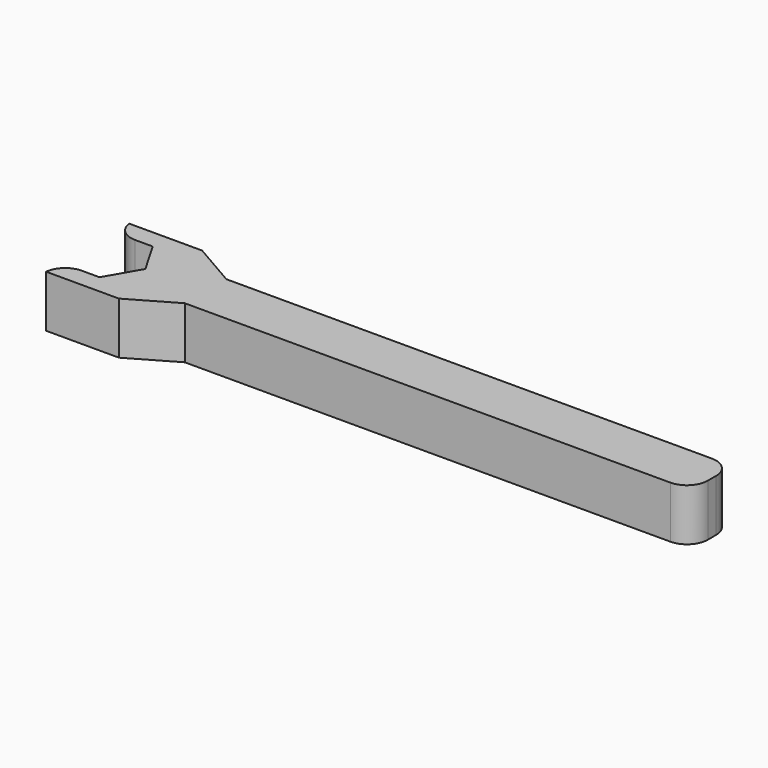
from build123d import *

# Parameters (mm, degrees)
F1_DEPTH    = 2.5
F2_T1_DEPTH = 14.9498743711
F2_T3_DEPTH = 15


# Not quite as in the source:
# - a fillet or chamfer that OpenCascade refuses, or shapes differently, is made with other operations: its cross-section is extruded or revolved along the edge and cut away or added


with BuildPart() as f1:
    # F0 (on Top) → F1 (new body, symmetric)
    with BuildSketch(Plane.XY):
        Polygon((1.8475208614, 3.2), (3.6950417228, 0), (1.8475208614, -3.2), (-1.8475208614, -3.2), (-1.8475208614, -5), (5.1524791386, -5), (9.4826061575, -2.5), (58.1524791386, -2.5), (58.1524791386, 2.5), (9.4826061575, 2.5), (5.1524791386, 5), (-1.8475208614, 5), (-1.8475208614, 3.2), align=None)
    extrude(amount=F1_DEPTH, both=True)

    # F2: fillet of radius 2 on 4 edges, made by hand

    # F2_s2 → F2_t1 (cut)
    with BuildSketch(Plane.XY.offset(-7.4749371855)):
        with BuildLine():
            ThreePointArc((-1.8475208614, 5), (-1.1991867737, 3.7167603026), (0.1424540128, 3.2))
            Line((0.1424540128, 3.2), (-1.8475208614, 3.2))
            Line((-1.8475208614, 3.2), (-1.8475208614, 5))
        make_face()
        with BuildLine():
            ThreePointArc((-1.8475208614, -5), (-1.1991867737, -3.7167603026), (0.1424540128, -3.2))
            Line((0.1424540128, -3.2), (-1.8475208614, -3.2))
            Line((-1.8475208614, -3.2), (-1.8475208614, -5))
        make_face()
    extrude(amount=F2_T1_DEPTH, mode=Mode.SUBTRACT)

    # F2_s4 → F2_t3 (cut)
    with BuildSketch(Plane.XY.offset(-7.5)):
        with BuildLine():
            ThreePointArc((58.1524791386, -0.5), (57.566692701, -1.9142135624), (56.1524791386, -2.5))
            Line((56.1524791386, -2.5), (58.1524791386, -2.5))
            Line((58.1524791386, -2.5), (58.1524791386, -0.5))
        make_face()
        with BuildLine():
            ThreePointArc((56.1524791386, 2.5), (57.566692701, 1.9142135624), (58.1524791386, 0.5))
            Line((58.1524791386, 0.5), (58.1524791386, 2.5))
            Line((58.1524791386, 2.5), (56.1524791386, 2.5))
        make_face()
    extrude(amount=F2_T3_DEPTH, mode=Mode.SUBTRACT)


solid = f1.part
